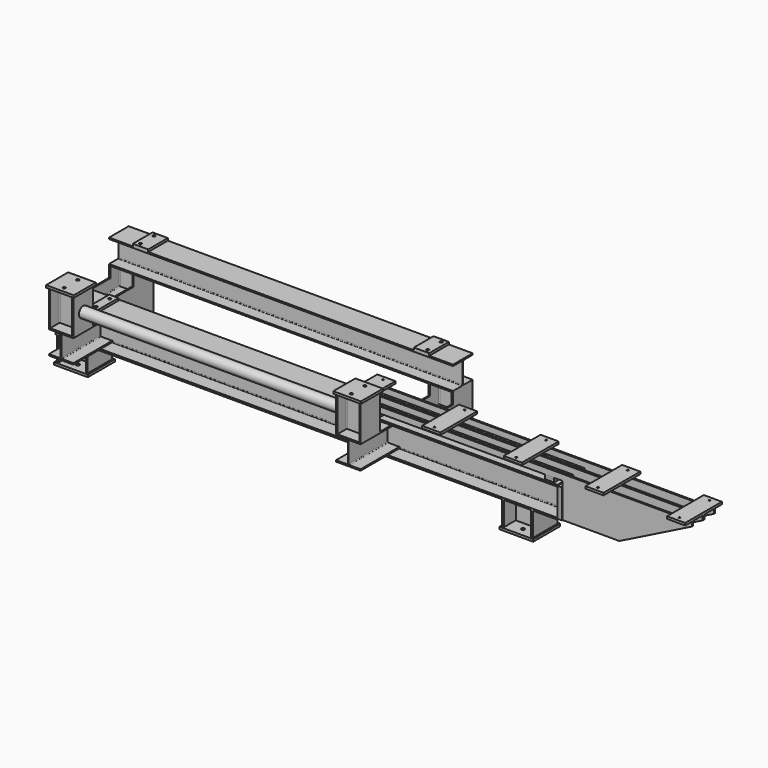
from build123d import *

# Parameters (mm, degrees)
F0_W        = 228.6
F0_H        = 228.6
F0_R        = 14.2875
F1_DEPTH    = 19.05
F0_W_2      = 279.4
F0_H_2      = 279.4
F3_DEPTH    = 504.952
F5_DEPTH    = 2844.8
F6_W        = 127
F6_H        = 203.2
F6_R        = 11.1125
F7_DEPTH    = 19.05
F9_DEPTH    = 482.6
F12_DEPTH   = 4152.9
F14_DEPTH   = 198.374
F15_W       = 76.2
F15_H       = 228.6
F15_R       = 11.1125
F16_DEPTH   = 19.05
F18_DEPTH   = 401.574
F20_DEPTH   = 292.1
F21_W       = 228.6
F21_H       = 228.6
F21_R       = 11.1125
F22_DEPTH   = 19.05
F23_R       = 44.45
F23_R_2     = 38.9636
F24_DEPTH   = 2171.7
F25_W       = 76.2
F25_H       = 228.6
F25_R       = 11.1125
F26_DEPTH   = 19
F28_W       = 150
F28_H       = 380
F28_R       = 7.25
F29_DEPTH   = 19
F31_W       = 254
F31_H       = 239.776
F31_R       = 10
F32_DEPTH   = 19
F33_W       = 254
F33_H       = 239.776
F33_R       = 10
F34_DEPTH   = 19
F36_DEPTH   = 9.5
F38_DEPTH   = 6.25
F39_SIZE2   = 600
F39_SIZE    = 300
F39_2_SIZE2 = 600
F39_2_SIZE  = 300
F41_SIZE    = 40
F41_2_SIZE  = 40
F41_3_SIZE  = 40


with BuildPart() as f1:
    # F0 (on Top) → F1 (new body)
    with BuildSketch(Plane.XY):
        with Locations((-1320.8, 241.3)):
            Rectangle(F0_W, F0_H)
        with Locations((-1320.8, 171.45)):
            Circle(F0_R, mode=Mode.SUBTRACT)
        with Locations((-1320.8, 311.15)):
            Circle(F0_R, mode=Mode.SUBTRACT)
    extrude(amount=F1_DEPTH)

    # F2 (on face) → F3 (join)
    with BuildSketch(Plane.XY.offset(19.05)):
        with BuildLine():
            Line((-1411.351, 342.9), (-1422.4, 342.9))
            Line((-1422.4, 342.9), (-1422.4, 139.7))
            Line((-1422.4, 139.7), (-1411.351, 139.7))
            Line((-1411.351, 139.7), (-1411.351, 231.3305))
            ThreePointArc((-1411.351, 231.3305), (-1409.4911280605, 235.8206280605), (-1405.001, 237.6805))
            Line((-1405.001, 237.6805), (-1320.8, 237.6805))
            Line((-1320.8, 237.6805), (-1236.599, 237.6805))
            ThreePointArc((-1236.599, 237.6805), (-1232.1088719395, 235.8206280605), (-1230.249, 231.3305))
            Line((-1230.249, 231.3305), (-1230.249, 139.7))
            Line((-1230.249, 139.7), (-1219.2, 139.7))
            Line((-1219.2, 139.7), (-1219.2, 342.9))
            Line((-1219.2, 342.9), (-1230.249, 342.9))
            Line((-1230.249, 342.9), (-1230.249, 251.2695))
            ThreePointArc((-1230.249, 251.2695), (-1232.1088719395, 246.7793719395), (-1236.599, 244.9195))
            Line((-1236.599, 244.9195), (-1320.8, 244.9195))
            Line((-1320.8, 244.9195), (-1405.001, 244.9195))
            ThreePointArc((-1405.001, 244.9195), (-1409.4911280605, 246.7793719395), (-1411.351, 251.2695))
            Line((-1411.351, 251.2695), (-1411.351, 342.9))
        make_face()
    extrude(amount=F3_DEPTH)



with BuildPart() as f1b:
    # F0 (on Top) → F1, piece 2 (new body)
    with BuildSketch(Plane.XY):
        with Locations((1320.8, 241.3)):
            Rectangle(F0_W, F0_H)
        with Locations((1320.8, 171.45)):
            Circle(F0_R, mode=Mode.SUBTRACT)
        with Locations((1320.8, 311.15)):
            Circle(F0_R, mode=Mode.SUBTRACT)
    extrude(amount=F1_DEPTH)

    # F2 (on face) → F3, piece 2 (join)
    with BuildSketch(Plane.XY.offset(19.05)):
        with BuildLine():
            Line((1411.351, 342.9), (1411.351, 251.2695))
            ThreePointArc((1411.351, 251.2695), (1409.4911280605, 246.7793719395), (1405.001, 244.9195))
            Line((1405.001, 244.9195), (1320.8, 244.9195))
            Line((1320.8, 244.9195), (1236.599, 244.9195))
            ThreePointArc((1236.599, 244.9195), (1232.1088719395, 246.7793719395), (1230.249, 251.2695))
            Line((1230.249, 251.2695), (1230.249, 342.9))
            Line((1230.249, 342.9), (1219.2, 342.9))
            Line((1219.2, 342.9), (1219.2, 139.7))
            Line((1219.2, 139.7), (1230.249, 139.7))
            Line((1230.249, 139.7), (1230.249, 231.3305))
            ThreePointArc((1230.249, 231.3305), (1232.1088719395, 235.8206280605), (1236.599, 237.6805))
            Line((1236.599, 237.6805), (1320.8, 237.6805))
            Line((1320.8, 237.6805), (1405.001, 237.6805))
            ThreePointArc((1405.001, 237.6805), (1409.4911280605, 235.8206280605), (1411.351, 231.3305))
            Line((1411.351, 231.3305), (1411.351, 139.7))
            Line((1411.351, 139.7), (1422.4, 139.7))
            Line((1422.4, 139.7), (1422.4, 342.9))
            Line((1422.4, 342.9), (1411.351, 342.9))
        make_face()
    extrude(amount=F3_DEPTH)


with BuildPart() as f1c:
    # F0 (on Top) → F1, piece 3 (new body)
    with BuildSketch(Plane.XY):
        with Locations((2362.2, -241.3)):
            Rectangle(F0_W_2, F0_H_2)
        with Locations((2362.2, -311.15)):
            Circle(F0_R, mode=Mode.SUBTRACT)
        with Locations((2362.2, -171.45)):
            Circle(F0_R, mode=Mode.SUBTRACT)
    extrude(amount=F1_DEPTH)


with BuildPart() as f1d:
    # F0 (on Top) → F1, piece 4 (new body)
    with BuildSketch(Plane.XY):
        with Locations((-1320.8, -241.3)):
            Rectangle(F0_W_2, F0_H_2)
        with Locations((-1320.8, -311.15)):
            Circle(F0_R, mode=Mode.SUBTRACT)
        with Locations((-1320.8, -171.45)):
            Circle(F0_R, mode=Mode.SUBTRACT)
    extrude(amount=F1_DEPTH)


with BuildPart() as f1_1:
    add(f1.part)

    add(f1b.part)  # F5 merges F1b
    # F4 (on face) → F5 (join, through all)
    with BuildSketch(Plane.YZ.offset(1422.4)):
        with BuildLine():
            Line((139.7, 535.051), (139.7, 524.002))
            Line((139.7, 524.002), (342.9, 524.002))
            Line((342.9, 524.002), (342.9, 535.051))
            Line((342.9, 535.051), (251.2695, 535.051))
            ThreePointArc((251.2695, 535.051), (246.7793719395, 536.9108719395), (244.9195, 541.401))
            Line((244.9195, 541.401), (244.9195, 709.803))
            ThreePointArc((244.9195, 709.803), (246.7793719395, 714.2931280605), (251.2695, 716.153))
            Line((251.2695, 716.153), (342.9, 716.153))
            Line((342.9, 716.153), (342.9, 727.202))
            Line((342.9, 727.202), (139.7, 727.202))
            Line((139.7, 727.202), (139.7, 716.153))
            Line((139.7, 716.153), (231.3305, 716.153))
            ThreePointArc((231.3305, 716.153), (235.8206280605, 714.2931280605), (237.6805, 709.803))
            Line((237.6805, 709.803), (237.6805, 541.401))
            ThreePointArc((237.6805, 541.401), (235.8206280605, 536.9108719395), (231.3305, 535.051))
            Line((231.3305, 535.051), (139.7, 535.051))
        make_face()
    extrude(amount=-F5_DEPTH)

    # F6 (on face) → F7 (join)
    with BuildSketch(Plane.XY.offset(727.202)):
        with Locations((1162.05, 241.3)):
            Rectangle(F6_W, F6_H)
        with Locations((1187.45, 171.45)):
            Circle(F6_R, mode=Mode.SUBTRACT)
        with Locations((1187.45, 311.15)):
            Circle(F6_R, mode=Mode.SUBTRACT)
        with Locations((-1162.05, 241.3)):
            Rectangle(F6_W, F6_H)
        with Locations((-1187.45, 171.45)):
            Circle(F6_R, mode=Mode.SUBTRACT)
        with Locations((-1187.45, 311.15)):
            Circle(F6_R, mode=Mode.SUBTRACT)
    extrude(amount=F7_DEPTH)

    # F8 (on face) → F9 (join)
    with BuildSketch(Plane.XZ.offset(-237.6805)):
        with BuildLine():
            Line((-1422.4, 434.848), (-1422.4, 231.648))
            Line((-1422.4, 231.648), (-1411.351, 231.648))
            Line((-1411.351, 231.648), (-1411.351, 328.803))
            ThreePointArc((-1411.351, 328.803), (-1410.9790256121, 329.7010256121), (-1410.081, 330.073))
            Line((-1410.081, 330.073), (-1320.8, 330.073))
            Line((-1320.8, 330.073), (-1231.519, 330.073))
            ThreePointArc((-1231.519, 330.073), (-1230.6209743879, 329.7010256121), (-1230.249, 328.803))
            Line((-1230.249, 328.803), (-1230.249, 231.648))
            Line((-1230.249, 231.648), (-1219.2, 231.648))
            Line((-1219.2, 231.648), (-1219.2, 434.848))
            Line((-1219.2, 434.848), (-1230.249, 434.848))
            Line((-1230.249, 434.848), (-1230.249, 342.773))
            ThreePointArc((-1230.249, 342.773), (-1232.1088719395, 338.2828719395), (-1236.599, 336.423))
            Line((-1236.599, 336.423), (-1320.8, 336.423))
            Line((-1320.8, 336.423), (-1405.001, 336.423))
            ThreePointArc((-1405.001, 336.423), (-1409.4911280605, 338.2828719395), (-1411.351, 342.773))
            Line((-1411.351, 342.773), (-1411.351, 434.848))
            Line((-1411.351, 434.848), (-1422.4, 434.848))
        make_face()
        with BuildLine():
            Line((1411.351, 434.848), (1411.351, 342.773))
            ThreePointArc((1411.351, 342.773), (1409.4911280605, 338.2828719395), (1405.001, 336.423))
            Line((1405.001, 336.423), (1320.8, 336.423))
            Line((1320.8, 336.423), (1236.599, 336.423))
            ThreePointArc((1236.599, 336.423), (1232.1088719395, 338.2828719395), (1230.249, 342.773))
            Line((1230.249, 342.773), (1230.249, 434.848))
            Line((1230.249, 434.848), (1219.2, 434.848))
            Line((1219.2, 434.848), (1219.2, 231.648))
            Line((1219.2, 231.648), (1230.249, 231.648))
            Line((1230.249, 231.648), (1230.249, 328.803))
            ThreePointArc((1230.249, 328.803), (1230.6209743879, 329.7010256121), (1231.519, 330.073))
            Line((1231.519, 330.073), (1320.8, 330.073))
            Line((1320.8, 330.073), (1410.081, 330.073))
            ThreePointArc((1410.081, 330.073), (1410.9790256121, 329.7010256121), (1411.351, 328.803))
            Line((1411.351, 328.803), (1411.351, 231.648))
            Line((1411.351, 231.648), (1422.4, 231.648))
            Line((1422.4, 231.648), (1422.4, 434.848))
            Line((1422.4, 434.848), (1411.351, 434.848))
        make_face()
    extrude(amount=F9_DEPTH)

    # F11 (on offset) → F12 (join)
    with BuildSketch(Plane.YZ.offset(2692.4)):
        with BuildLine():
            Line((-368.3, 231.648), (-368.3, 217.424))
            Line((-368.3, 217.424), (-114.3, 217.424))
            Line((-114.3, 217.424), (-114.3, 231.648))
            Line((-114.3, 231.648), (-228.6, 231.648))
            ThreePointArc((-228.6, 231.648), (-233.0901280605, 233.5078719395), (-234.95, 237.998))
            Line((-234.95, 237.998), (-234.95, 450.85))
            ThreePointArc((-234.95, 450.85), (-233.0901280605, 455.3401280605), (-228.6, 457.2))
            Line((-228.6, 457.2), (-114.3, 457.2))
            Line((-114.3, 457.2), (-114.3, 471.424))
            Line((-114.3, 471.424), (-368.3, 471.424))
            Line((-368.3, 471.424), (-368.3, 457.2))
            Line((-368.3, 457.2), (-254, 457.2))
            ThreePointArc((-254, 457.2), (-249.5098719395, 455.3401280605), (-247.65, 450.85))
            Line((-247.65, 450.85), (-247.65, 237.998))
            ThreePointArc((-247.65, 237.998), (-249.5098719395, 233.5078719395), (-254, 231.648))
            Line((-254, 231.648), (-368.3, 231.648))
        make_face()
    extrude(amount=-F12_DEPTH)


    add(f1c.part)  # F14 merges F1c

    add(f1d.part)  # F14 merges F1d
    # F13 (on face) → F14 (join)
    with BuildSketch(Plane.XY.offset(19.05)):
        Polygon((-1433.576, -114.3), (-1447.8, -114.3), (-1447.8, -368.3), (-1433.576, -368.3), (-1433.576, -245.618), (-1208.024, -245.618), (-1208.024, -368.3), (-1193.8, -368.3), (-1193.8, -114.3), (-1208.024, -114.3), (-1208.024, -236.982), (-1433.576, -236.982), align=None)
        Polygon((2474.976, -368.3), (2489.2, -368.3), (2489.2, -114.3), (2474.976, -114.3), (2474.976, -236.982), (2249.424, -236.982), (2249.424, -114.3), (2235.2, -114.3), (2235.2, -368.3), (2249.424, -368.3), (2249.424, -245.618), (2474.976, -245.618), align=None)
    extrude(amount=F14_DEPTH)

    # F15 (on face) → F16 (join)
    with BuildSketch(Plane.XY.offset(471.424)):
        with Locations((-1168.4, -241.3)):
            Rectangle(F15_W, F15_H)
        with Locations((-1168.4, -311.15)):
            Circle(F15_R, mode=Mode.SUBTRACT)
        with Locations((-1168.4, -171.45)):
            Circle(F15_R, mode=Mode.SUBTRACT)
        with Locations((1168.4, -241.3)):
            Rectangle(F15_W, F15_H)
        with Locations((1168.4, -311.15)):
            Circle(F15_R, mode=Mode.SUBTRACT)
        with Locations((1168.4, -171.45)):
            Circle(F15_R, mode=Mode.SUBTRACT)
        with Locations((2616.2, -241.3)):
            Rectangle(F15_W, F15_H)
        with Locations((2616.2, -311.15)):
            Circle(F15_R, mode=Mode.SUBTRACT)
        with Locations((2616.2, -171.45)):
            Circle(F15_R, mode=Mode.SUBTRACT)
    extrude(amount=F16_DEPTH)

    # F17 (on face) → F18 (join)
    with BuildSketch(Plane.XZ.offset(247.65)):
        with BuildLine():
            Line((-1085.85, 435.102), (-1289.05, 435.102))
            Line((-1289.05, 435.102), (-1289.05, 424.053))
            Line((-1289.05, 424.053), (-1197.356, 424.053))
            ThreePointArc((-1197.356, 424.053), (-1192.8658719395, 422.1931280605), (-1191.006, 417.703))
            Line((-1191.006, 417.703), (-1191.006, 249.301))
            ThreePointArc((-1191.006, 249.301), (-1192.8658719395, 244.8108719395), (-1197.356, 242.951))
            Line((-1197.356, 242.951), (-1289.05, 242.951))
            Line((-1289.05, 242.951), (-1289.05, 231.902))
            Line((-1289.05, 231.902), (-1085.85, 231.902))
            Line((-1085.85, 231.902), (-1085.85, 242.951))
            Line((-1085.85, 242.951), (-1177.544, 242.951))
            ThreePointArc((-1177.544, 242.951), (-1182.0341280605, 244.8108719395), (-1183.894, 249.301))
            Line((-1183.894, 249.301), (-1183.894, 417.703))
            ThreePointArc((-1183.894, 417.703), (-1182.0341280605, 422.1931280605), (-1177.544, 424.053))
            Line((-1177.544, 424.053), (-1085.85, 424.053))
            Line((-1085.85, 424.053), (-1085.85, 435.102))
        make_face()
        with BuildLine():
            Line((1085.85, 424.053), (1177.544, 424.053))
            ThreePointArc((1177.544, 424.053), (1182.0341280605, 422.1931280605), (1183.894, 417.703))
            Line((1183.894, 417.703), (1183.894, 249.301))
            ThreePointArc((1183.894, 249.301), (1182.0341280605, 244.8108719395), (1177.544, 242.951))
            Line((1177.544, 242.951), (1085.85, 242.951))
            Line((1085.85, 242.951), (1085.85, 231.902))
            Line((1085.85, 231.902), (1289.05, 231.902))
            Line((1289.05, 231.902), (1289.05, 242.951))
            Line((1289.05, 242.951), (1197.356, 242.951))
            ThreePointArc((1197.356, 242.951), (1192.8658719395, 244.8108719395), (1191.006, 249.301))
            Line((1191.006, 249.301), (1191.006, 417.703))
            ThreePointArc((1191.006, 417.703), (1192.8658719395, 422.1931280605), (1197.356, 424.053))
            Line((1197.356, 424.053), (1289.05, 424.053))
            Line((1289.05, 424.053), (1289.05, 435.102))
            Line((1289.05, 435.102), (1085.85, 435.102))
            Line((1085.85, 435.102), (1085.85, 424.053))
        make_face()
    extrude(amount=F18_DEPTH)

    # F19 (on face) → F20 (join)
    with BuildSketch(Plane.XY.offset(435.102)):
        with BuildLine():
            Line((-1289.05, -446.024), (-1289.05, -649.224))
            Line((-1289.05, -649.224), (-1278.001, -649.224))
            Line((-1278.001, -649.224), (-1278.001, -557.53))
            ThreePointArc((-1278.001, -557.53), (-1276.1411280605, -553.0398719395), (-1271.651, -551.18))
            Line((-1271.651, -551.18), (-1103.249, -551.18))
            ThreePointArc((-1103.249, -551.18), (-1098.7588719395, -553.0398719395), (-1096.899, -557.53))
            Line((-1096.899, -557.53), (-1096.899, -649.224))
            Line((-1096.899, -649.224), (-1085.85, -649.224))
            Line((-1085.85, -649.224), (-1085.85, -446.024))
            Line((-1085.85, -446.024), (-1096.899, -446.024))
            Line((-1096.899, -446.024), (-1096.899, -537.718))
            ThreePointArc((-1096.899, -537.718), (-1098.7588719395, -542.2081280605), (-1103.249, -544.068))
            Line((-1103.249, -544.068), (-1271.651, -544.068))
            ThreePointArc((-1271.651, -544.068), (-1276.1411280605, -542.2081280605), (-1278.001, -537.718))
            Line((-1278.001, -537.718), (-1278.001, -446.024))
            Line((-1278.001, -446.024), (-1289.05, -446.024))
        make_face()
        with BuildLine():
            Line((1103.249, -551.18), (1271.651, -551.18))
            ThreePointArc((1271.651, -551.18), (1276.1411280605, -553.0398719395), (1278.001, -557.53))
            Line((1278.001, -557.53), (1278.001, -649.224))
            Line((1278.001, -649.224), (1289.05, -649.224))
            Line((1289.05, -649.224), (1289.05, -446.024))
            Line((1289.05, -446.024), (1278.001, -446.024))
            Line((1278.001, -446.024), (1278.001, -537.718))
            ThreePointArc((1278.001, -537.718), (1276.1411280605, -542.2081280605), (1271.651, -544.068))
            Line((1271.651, -544.068), (1103.249, -544.068))
            ThreePointArc((1103.249, -544.068), (1098.7588719395, -542.2081280605), (1096.899, -537.718))
            Line((1096.899, -537.718), (1096.899, -446.024))
            Line((1096.899, -446.024), (1085.85, -446.024))
            Line((1085.85, -446.024), (1085.85, -649.224))
            Line((1085.85, -649.224), (1096.899, -649.224))
            Line((1096.899, -649.224), (1096.899, -557.53))
            ThreePointArc((1096.899, -557.53), (1098.7588719395, -553.0398719395), (1103.249, -551.18))
        make_face()
    extrude(amount=F20_DEPTH)

    # F21 (on face) → F22 (join)
    with BuildSketch(Plane.XY.offset(727.202)):
        with Locations((-1187.45, -547.624)):
            Rectangle(F21_W, F21_H)
        with Locations((-1187.45, -617.474)):
            Circle(F21_R, mode=Mode.SUBTRACT)
        with Locations((-1187.45, -477.774)):
            Circle(F21_R, mode=Mode.SUBTRACT)
        with Locations((1187.45, -547.624)):
            Rectangle(F21_W, F21_H)
        with Locations((1187.45, -617.474)):
            Circle(F21_R, mode=Mode.SUBTRACT)
        with Locations((1187.45, -477.774)):
            Circle(F21_R, mode=Mode.SUBTRACT)
    extrude(amount=F22_DEPTH)

    # F23 (on face) → F24 (join)
    with BuildSketch(Plane.YZ.offset(-1085.85)):
        with Locations((-547.624, 574.802)):
            Circle(F23_R)
        with Locations((-547.624, 574.802)):
            Circle(F23_R_2, mode=Mode.SUBTRACT)
    extrude(amount=F24_DEPTH)


with BuildPart() as f26:
    # F25 (on face) → F26 (new body)
    with BuildSketch(Plane.XY.offset(490.474)):
        with Locations((1168.4, -241.3)):
            Rectangle(F25_W, F25_H)
        with Locations((1168.4, -311.15)):
            Circle(F25_R, mode=Mode.SUBTRACT)
        with Locations((1168.4, -171.45)):
            Circle(F25_R, mode=Mode.SUBTRACT)
    extrude(amount=F26_DEPTH)


with BuildPart() as f26b:
    # F25 (on face) → F26, piece 2 (new body)
    with BuildSketch(Plane.XY.offset(490.474)):
        with Locations((2616.2, -241.3)):
            Rectangle(F25_W, F25_H)
        with Locations((2616.2, -311.15)):
            Circle(F25_R, mode=Mode.SUBTRACT)
        with Locations((2616.2, -171.45)):
            Circle(F25_R, mode=Mode.SUBTRACT)
    extrude(amount=F26_DEPTH)


with BuildPart() as f29:
    # F28 (on offset) → F29 (new body)
    with BuildSketch(Plane.XY.offset(579.424)):
        with Locations((1023.9, -241.3)):
            Rectangle(F28_W, F28_H)
        with Locations((1023.9, -396.3)):
            Circle(F28_R, mode=Mode.SUBTRACT)
        with Locations((1023.9, -86.3)):
            Circle(F28_R, mode=Mode.SUBTRACT)
    extrude(amount=-F29_DEPTH)


with BuildPart() as f29b:
    # F28 (on offset) → F29, piece 2 (new body)
    with BuildSketch(Plane.XY.offset(579.424)):
        with Locations((1698.9, -241.3)):
            Rectangle(F28_W, F28_H)
        with Locations((1698.9, -396.3)):
            Circle(F28_R, mode=Mode.SUBTRACT)
        with Locations((1698.9, -86.3)):
            Circle(F28_R, mode=Mode.SUBTRACT)
    extrude(amount=-F29_DEPTH)


with BuildPart() as f29c:
    # F28 (on offset) → F29, piece 3 (new body)
    with BuildSketch(Plane.XY.offset(579.424)):
        with Locations((2373.9, -241.3)):
            Rectangle(F28_W, F28_H)
        with Locations((2373.9, -396.3)):
            Circle(F28_R, mode=Mode.SUBTRACT)
        with Locations((2373.9, -86.3)):
            Circle(F28_R, mode=Mode.SUBTRACT)
    extrude(amount=-F29_DEPTH)


with BuildPart() as f29d:
    # F28 (on offset) → F29, piece 4 (new body)
    with BuildSketch(Plane.XY.offset(579.424)):
        with Locations((3048.9, -241.3)):
            Rectangle(F28_W, F28_H)
        with Locations((3048.9, -396.3)):
            Circle(F28_R, mode=Mode.SUBTRACT)
        with Locations((3048.9, -86.3)):
            Circle(F28_R, mode=Mode.SUBTRACT)
    extrude(amount=-F29_DEPTH)


with BuildPart() as f29e:
    # F28 (on offset) → F29, piece 5 (new body)
    with BuildSketch(Plane.XY.offset(579.424)):
        with Locations((3723.9, -241.3)):
            Rectangle(F28_W, F28_H)
        with Locations((3723.9, -396.3)):
            Circle(F28_R, mode=Mode.SUBTRACT)
        with Locations((3723.9, -86.3)):
            Circle(F28_R, mode=Mode.SUBTRACT)
    extrude(amount=-F29_DEPTH)


with BuildPart() as f32:
    # F31 (on offset) → F32 (new body)
    with BuildSketch(Plane.YZ.offset(2692.4)):
        with Locations((-241.3, 344.424)):
            Rectangle(F31_W, F31_H)
        with Locations((-328.3, 264.424)):
            Circle(F31_R, mode=Mode.SUBTRACT)
        with Locations((-328.3, 344.424)):
            Circle(F31_R, mode=Mode.SUBTRACT)
        with Locations((-154.3, 264.424)):
            Circle(F31_R, mode=Mode.SUBTRACT)
        with Locations((-154.3, 344.424)):
            Circle(F31_R, mode=Mode.SUBTRACT)
        with Locations((-328.3, 424.424)):
            Circle(F31_R, mode=Mode.SUBTRACT)
        with Locations((-154.3, 424.424)):
            Circle(F31_R, mode=Mode.SUBTRACT)
    extrude(amount=F32_DEPTH)


with BuildPart() as f34:
    # F33 (on face) → F34 (new body)
    with BuildSketch(Plane.YZ.offset(2711.4)):
        with Locations((-241.3, 344.424)):
            Rectangle(F33_W, F33_H)
        with Locations((-328.3, 264.424)):
            Circle(F33_R, mode=Mode.SUBTRACT)
        with Locations((-328.3, 344.424)):
            Circle(F33_R, mode=Mode.SUBTRACT)
        with Locations((-154.3, 264.424)):
            Circle(F33_R, mode=Mode.SUBTRACT)
        with Locations((-154.3, 344.424)):
            Circle(F33_R, mode=Mode.SUBTRACT)
        with Locations((-328.3, 424.424)):
            Circle(F33_R, mode=Mode.SUBTRACT)
        with Locations((-154.3, 424.424)):
            Circle(F33_R, mode=Mode.SUBTRACT)
    extrude(amount=F34_DEPTH)


with BuildPart() as f36:
    # F35 (on mid) → F36 (new body, symmetric)
    with BuildSketch(Plane.XZ.offset(241.3)):
        with BuildLine():
            Line((3798.9, 560.424), (948.9, 560.424))
            Line((948.9, 560.424), (948.9, 509.474))
            Line((948.9, 509.474), (2720.4, 509.474))
            ThreePointArc((2720.4, 509.474), (2727.4710678119, 506.5450678119), (2730.4, 499.474))
            Line((2730.4, 499.474), (2730.4, 464.312))
            Line((2730.4, 464.312), (2730.4, 224.536))
            Line((2730.4, 224.536), (3798.9, 224.536))
            Line((3798.9, 224.536), (3798.9, 560.424))
        make_face()
    extrude(amount=F36_DEPTH, both=True)

    # F39
    f39_edges = [f36.edges().sort_by_distance(p)[0] for p in [
        (3798.9, -241.3, 224.536),
    ]]
    f39_side = f36.faces().sort_by_distance((3798.9, -241.3, 392.48))[0]
    chamfer(f39_edges, length=F39_SIZE, length2=F39_SIZE2, reference=f39_side)

    # F41
    f41_edges = [f36.edges().sort_by_distance(p)[0] for p in [
        (948.9, -241.3, 509.474),
    ]]
    chamfer(f41_edges, length=F41_SIZE)


with BuildPart() as f38:
    # F37 (on face) → F38 (new body, symmetric)
    with BuildSketch(Plane.XZ.offset(355.6)):
        with BuildLine():
            Line((3798.9, 224.536), (3798.9, 560.424))
            Line((3798.9, 560.424), (948.9, 560.424))
            Line((948.9, 560.424), (948.9, 509.474))
            Line((948.9, 509.474), (2720.4, 509.474))
            ThreePointArc((2720.4, 509.474), (2727.4710678119, 506.5450678119), (2730.4, 499.474))
            Line((2730.4, 499.474), (2730.4, 224.536))
            Line((2730.4, 224.536), (3798.9, 224.536))
        make_face()
    extrude(amount=F38_DEPTH, both=True)

    # F39#2
    f39_2_edges = [f38.edges().sort_by_distance(p)[0] for p in [
        (3798.9, -355.6, 224.536),
    ]]
    f39_2_side = f38.faces().sort_by_distance((3798.9, -355.6, 392.48))[0]
    chamfer(f39_2_edges, length=F39_2_SIZE, length2=F39_2_SIZE2, reference=f39_2_side)


with BuildPart() as f40_1:
    # F40: instance of F38
    add(f38.part.mirror(Plane(origin=(1168.4, -241.3, 499.974), x_dir=(1, 0, 0), z_dir=(0, -1, 0))))

    # F41#3
    f41_3_edges = [f40_1.edges().sort_by_distance(p)[0] for p in [
        (948.9, -127, 509.474),
    ]]
    chamfer(f41_3_edges, length=F41_3_SIZE)


with BuildPart() as f38_1:
    add(f38.part)

    # F41#2
    f41_2_edges = [f38_1.edges().sort_by_distance(p)[0] for p in [
        (948.9, -355.6, 509.474),
    ]]
    chamfer(f41_2_edges, length=F41_2_SIZE)


solid = Compound([f1_1.part, f26.part, f26b.part, f29.part, f29b.part, f29c.part, f29d.part, f29e.part, f32.part, f34.part, f36.part, f40_1.part, f38_1.part])
